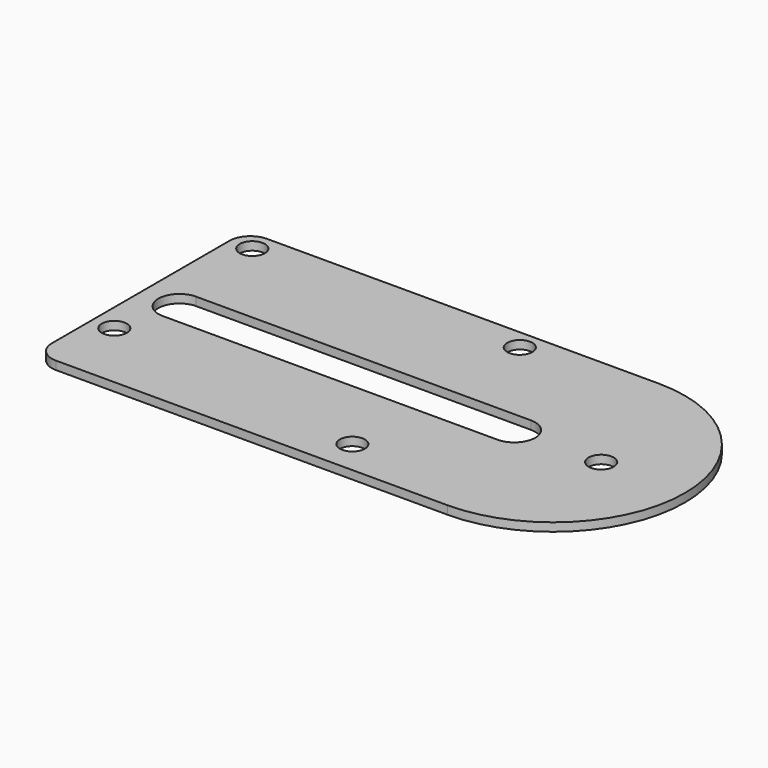
from build123d import *

# Parameters (mm, degrees)
F1_DEPTH = 2
F2_D     = 6
F3_R     = 5


with BuildPart() as f1:
    # F0 (on Top) → F1 (new body)
    with BuildSketch(Plane.XY):
        with BuildLine():
            Line((0, 31.5), (-98.5, 31.5))
            Line((-98.5, 31.5), (-98.5, -31.5))
            Line((-98.5, -31.5), (0, -31.5))
            ThreePointArc((0, -31.5), (31.5, 0), (0, 31.5))
        make_face()
        with BuildLine():
            Line((-9.25, -5), (-89.25, -5))
            ThreePointArc((-89.25, -5), (-94.25, 0), (-89.25, 5))
            Line((-89.25, 5), (-9.25, 5))
            ThreePointArc((-9.25, 5), (-4.25, 0), (-9.25, -5))
        make_face(mode=Mode.SUBTRACT)
    extrude(amount=F1_DEPTH)

    # F2 (through all)
    with Locations(Plane(origin=(0, 0, 0), x_dir=(1, 0, 0), z_dir=(0, 0, -1))):
        with Locations((-93.2, -26.7), (-93.2, 14.5), (-29.3, -26.7), (-29.3, 23.3), (11.5, 0)):
            Hole(F2_D / 2)

    # F3
    f3_edges = [f1.edges().sort_by_distance(p)[0] for p in [
        (-98.5, 31.5, 1),
        (-98.5, -31.5, 1),
    ]]
    fillet(f3_edges, radius=F3_R)


solid = f1.part
